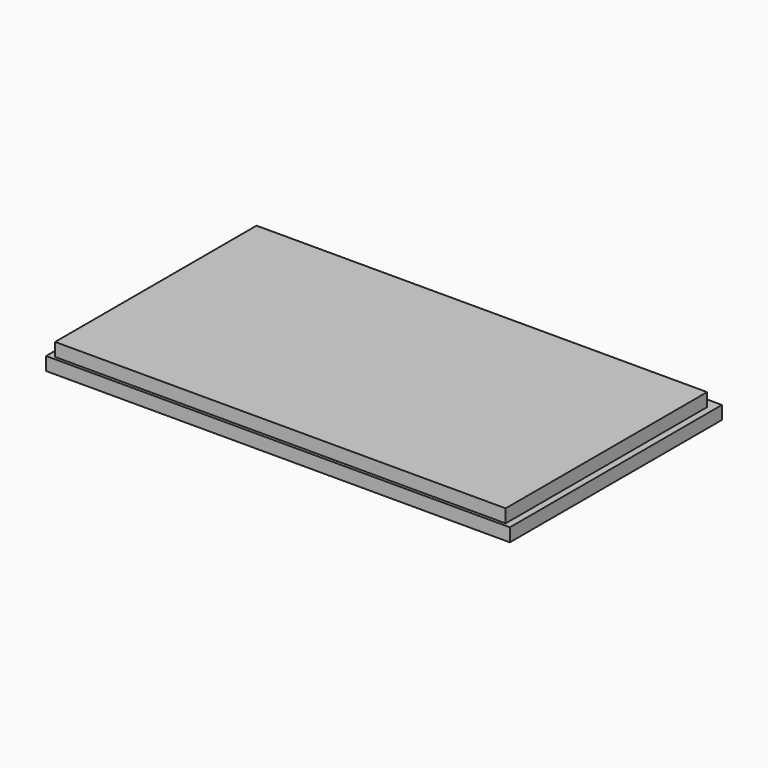
from build123d import *

# Parameters (mm, degrees)
F0_W         = 12.7
F0_H         = 50.8
F0_W_2       = 76.2
F1_DEPTH     = 2.54
F2_W         = 86.36
F2_H         = 48.26
F3_DEPTH     = 5.08
F4_TEXT_SIZE = 28.1611703233
F5_DEPTH     = 2.54


# Not quite as in the source:
# - Text() gives the source's letters only with a copy of the font that has no kerning and outlines rounded to 1/6400 em; it was checked with that copy


with BuildPart() as f1:
    # F0 (on Top) → F1 (new body)
    with BuildSketch(Plane.XY):
        with Locations((-74.4453929365, 5.6432374033)):
            Rectangle(F0_W, F0_H)
        with Locations((-29.9953929365, 5.6432374033)):
            Rectangle(F0_W_2, F0_H)
    extrude(amount=F1_DEPTH)

    # F2 (on Top) → F3 (join)
    with BuildSketch(Plane.XY):
        with Locations((-36.3621050492, 4.970480507)):
            Rectangle(F2_W, F2_H)
    extrude(amount=F3_DEPTH)

    # F4 (on Top) → F5 (join)
    with BuildSketch(Plane.XY):
        with Locations((-67.3920214176, -6.5802941099)):
            Text('john', F4_TEXT_SIZE, font='Open Sans', font_style=FontStyle.BOLD, text_align=(TextAlign.LEFT, TextAlign.BOTTOM))
    extrude(amount=-F5_DEPTH)


solid = f1.part
